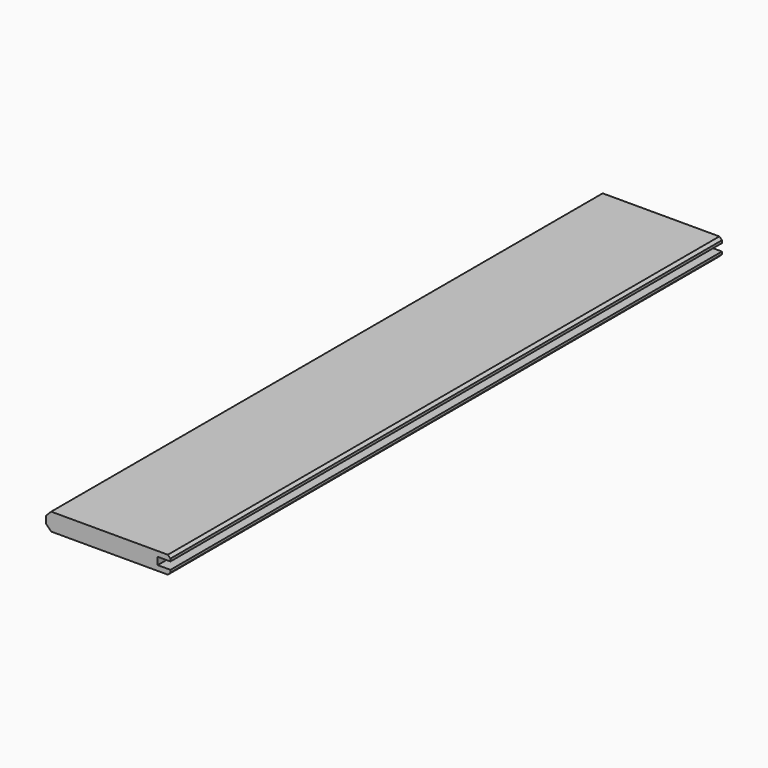
from build123d import *

# Parameters (mm, degrees)
F1_DEPTH = 685.8
F2_SIZE  = 2.54
F3_SIZE  = 5.07999
F4_W     = 25.4
F4_H     = 7.3152
F5_DEPTH = 685.801


# Not quite as in the source:
# - a fillet or chamfer is up to 0.001 mm smaller than in the source, because OpenCascade refuses the exact size


with BuildPart() as f1:
    # F0 (on Front) → F1 (new body)
    with BuildSketch(Plane.XZ):
        Polygon((68.199, 3.6576), (68.199, 8.7376), (-55.499, 8.7376), (-55.499, 3.6576), (-68.199, 3.6576), (-68.199, -3.6576), (-55.499, -3.6576), (-55.499, -8.7376), (68.199, -8.7376), (68.199, -3.6576), (55.499, -3.6576), (55.499, 3.6576), align=None)
    extrude(amount=F1_DEPTH)

    # F2
    f2_edges = [f1.edges().sort_by_distance(p)[0] for p in [
        (68.199, -342.9, 8.7376),
        (68.199, -342.9, -8.7376),
        (-68.199, -342.9, 3.6576),
        (-68.199, -342.9, -3.6576),
    ]]
    chamfer(f2_edges, length=F2_SIZE)

    # F3 (size 5.08 in the source; OpenCascade refuses exactly that, so slightly less here)
    f3_edges = [f1.edges().sort_by_distance(p)[0] for p in [
        (-55.499, -342.9, 8.7376),
        (-55.499, -342.9, -8.7376),
    ]]
    chamfer(f3_edges, length=F3_SIZE)

    # F4 (on face) → F5 (cut, through all)
    with BuildSketch(Plane.XZ.offset(685.8)):
        with Locations((-68.199, 0)):
            Rectangle(F4_W, F4_H)
    extrude(amount=-F5_DEPTH, mode=Mode.SUBTRACT)


solid = f1.part
